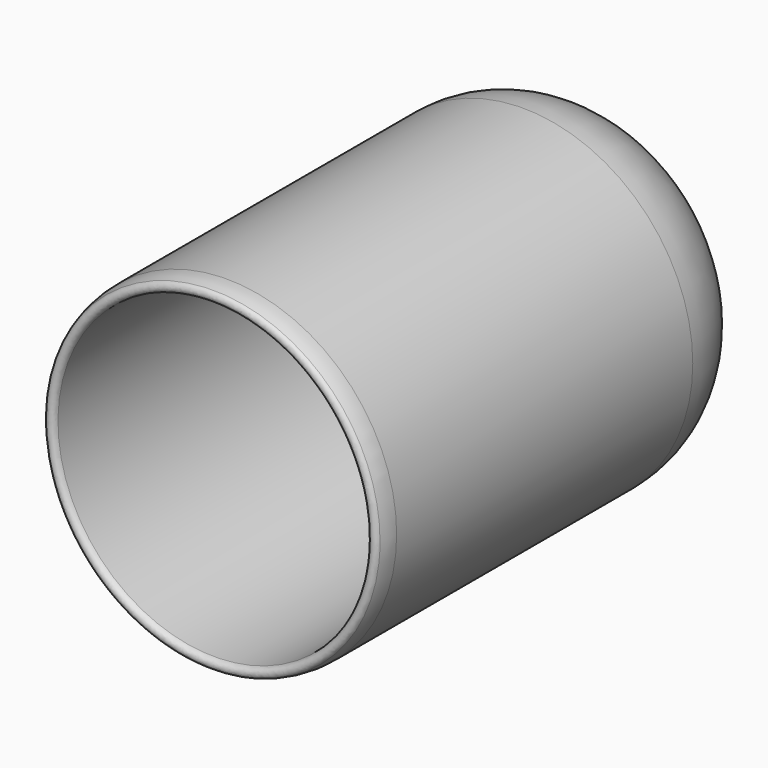
from build123d import *

# Parameters (mm, degrees)
F0_R     = 41.275
F1_DEPTH = 123.825
F2_R     = 38.1
F3_DEPTH = 114.3
F5_R     = 1.27
F6_R     = 25.4


# Not quite as in the source:
# - a fillet or chamfer that OpenCascade refuses, or shapes differently, is made with other operations: its cross-section is extruded or revolved along the edge and cut away or added


with BuildPart() as f1:
    # F0 (on Front) → F1 (new body)
    with BuildSketch(Plane.XZ):
        Circle(F0_R)
    extrude(amount=F1_DEPTH)

    # F2 (on face) → F3 (cut)
    with BuildSketch(Plane.XZ.offset(123.825)):
        Circle(F2_R)
    extrude(amount=-F3_DEPTH, mode=Mode.SUBTRACT)

    # F4: fillet of radius 12.7 on 2 edges, made by hand

    # F4_s1 → F4_t2 (revolve)
    with BuildSketch(Plane.XY):
        with BuildLine():
            ThreePointArc((38.1, -22.225), (34.3802561211, -13.2447438789), (25.4, -9.525))
            Line((25.4, -9.525), (38.1, -9.525))
            Line((38.1, -9.525), (38.1, -22.225))
        make_face()
    revolve(axis=Axis((0, -9.525, 0), (0, -1, 0)))

    # F4_s3 → F4_t4 (revolve, cut)
    with BuildSketch(Plane.XY):
        with BuildLine():
            ThreePointArc((41.275, -115.4247395874), (40.454762203, -119.9148676479), (38.1, -123.825))
            Line((38.1, -123.825), (41.275, -123.825))
            Line((41.275, -123.825), (41.275, -115.4247395874))
        make_face()
    revolve(axis=Axis((0, -123.825, 0), (0, -1, 0)), mode=Mode.SUBTRACT)

    # F5
    f5_edges = [f1.edges().sort_by_distance(p)[0] for p in [
        (-38.1, -123.825, 0),
    ]]
    fillet(f5_edges, radius=F5_R)

    # F6
    f6_edges = [f1.edges().sort_by_distance(p)[0] for p in [
        (-41.275, 0, 0),
    ]]
    fillet(f6_edges, radius=F6_R)


solid = f1.part
